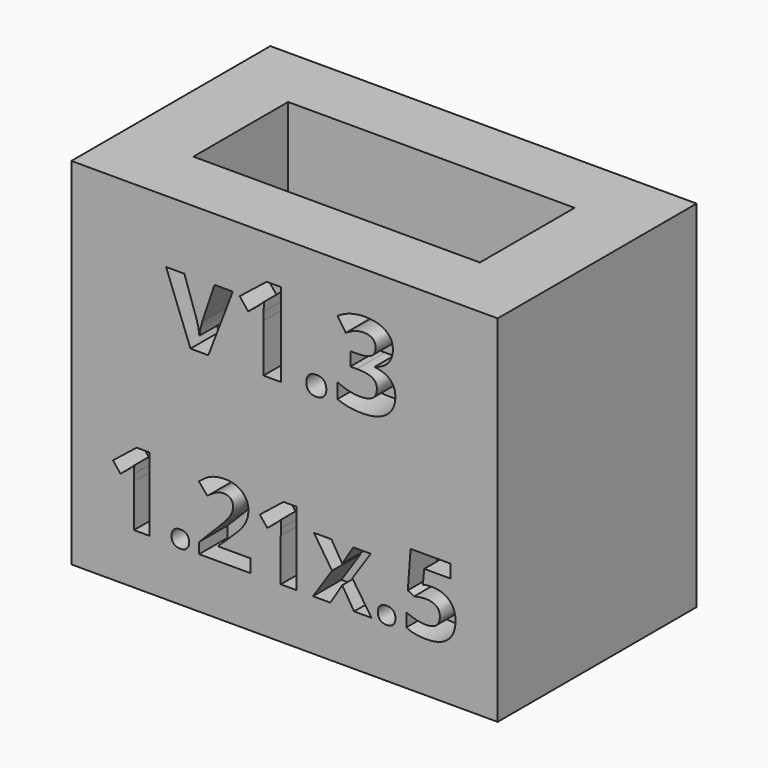
from build123d import *

# Parameters (mm, degrees)
F0_W           = 18
F0_H           = 10.5
F1_DEPTH       = 7.5
F2_W           = 12.1
F2_H           = 5
F3_DEPTH       = 13.5
F4_TEXT_SIZE   = 4.9459041731
F4_TEXT_SIZE_2 = 4.3458578542
F5_DEPTH       = 1.5


# Not quite as in the source:
# - Text() gives the source's letters only with a copy of the font that has no kerning and outlines rounded to 1/6400 em; it was checked with that copy


with BuildPart() as f1:
    # F0 (on Top) → F1 (new body, symmetric)
    with BuildSketch(Plane.XY):
        Rectangle(F0_W, F0_H)
    extrude(amount=F1_DEPTH, both=True)

    # F2 (on face) → F3 (cut)
    with BuildSketch(Plane.XY.offset(7.5)):
        Rectangle(F2_W, F2_H)
    extrude(amount=-F3_DEPTH, mode=Mode.SUBTRACT)

    # F4 (on face) → F5 (cut)
    with BuildSketch(Plane.XZ.offset(5.25)):
        with Locations((-5, 2.1578216251)):
            Text('v1.3', F4_TEXT_SIZE, font='Open Sans', font_style=FontStyle.BOLD, text_align=(TextAlign.LEFT, TextAlign.BOTTOM))
        with Locations((-7.5, -5.3649998729)):
            Text('1.21x.5', F4_TEXT_SIZE_2, font='Open Sans', font_style=FontStyle.BOLD, text_align=(TextAlign.LEFT, TextAlign.BOTTOM))
    extrude(amount=-F5_DEPTH, mode=Mode.SUBTRACT)


solid = f1.part
